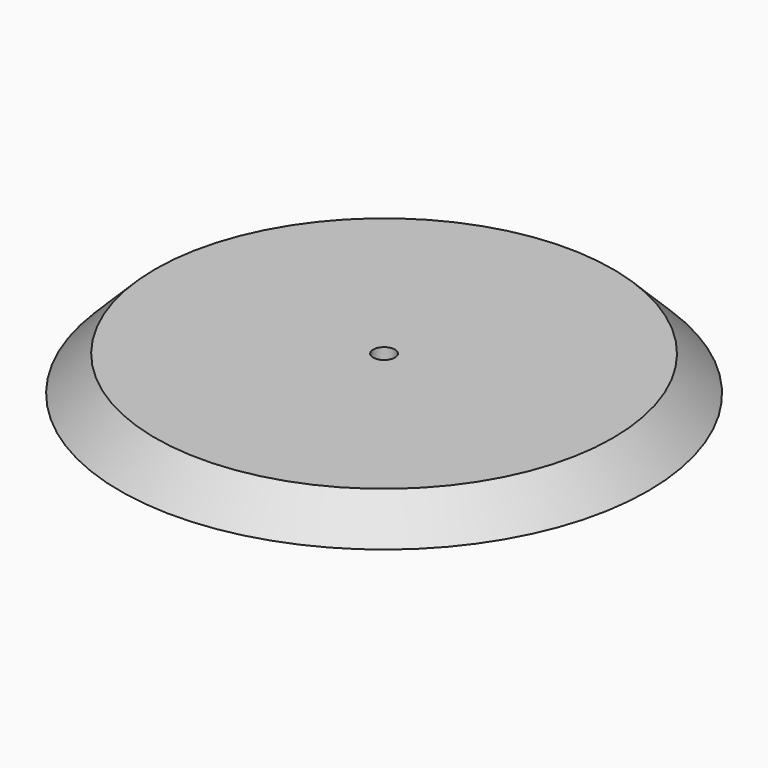
from build123d import *

# Parameters (mm, degrees)
F0_R     = 31.75
F1_DEPTH = 4.1021592915
F5_D     = 2.54


# Not quite as in the source:
# - a fillet or chamfer that OpenCascade refuses, or shapes differently, is made with other operations: its cross-section is extruded or revolved along the edge and cut away or added
# - the program builds the solid bodies; features that only make, move or delete a surface that nothing else refers to are left out


with BuildPart() as f1:
    # F0 (on Top) → F1 (new body)
    with BuildSketch(Plane.XY):
        Circle(F0_R)
    extrude(amount=F1_DEPTH)

    # F2: chamfer of 5.08 on 1 edges, made by hand

    # F2_s1 → F2_t2 (revolve, cut)
    with BuildSketch(Plane.XZ):
        Polygon((31.75, -0.9778407085), (26.67, 4.1021592915), (31.75, 4.1021592915), align=None)
    revolve(axis=Axis((0, 0, 4.1021592915), (0, 0, 1)), mode=Mode.SUBTRACT)

    # F5 (through all)
    with Locations(Plane.XY.offset(4.1021592915)):
        with Locations((0, 0)):
            Hole(F5_D / 2)


solid = f1.part
